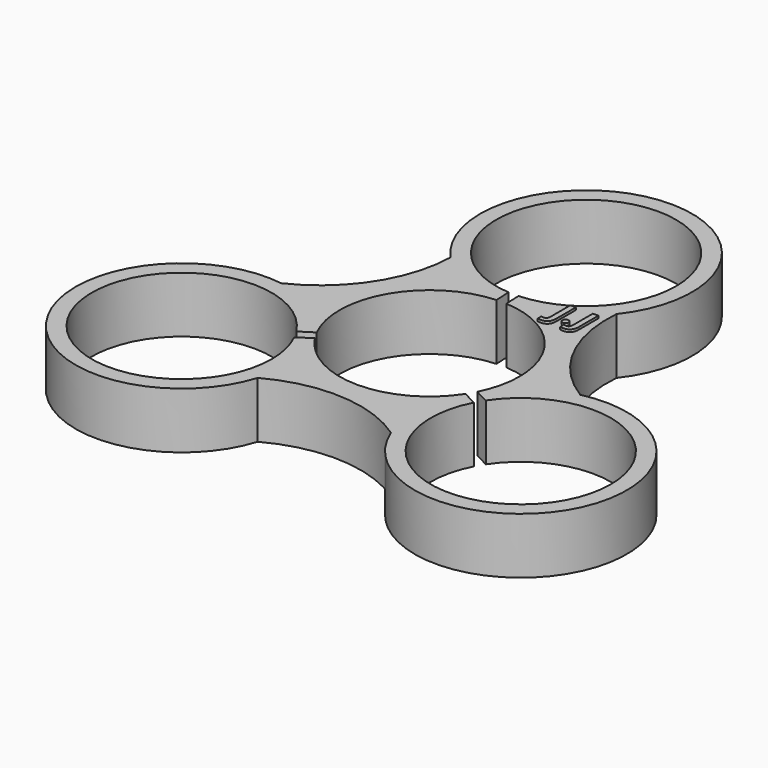
from build123d import *

# Parameters (mm, degrees)
F1_DEPTH     = 7
F2_TEXT_SIZE = 4.5465331318
F3_DEPTH     = 0.3


# Not quite as in the source:
# - Text() gives the source's letters only with a copy of the font that has no kerning and outlines rounded to 1/6400 em; it was checked with that copy


with BuildPart() as f1:
    # F0 (on Top) → F1 (new body)
    with BuildSketch(Plane.XY):
        with BuildLine():
            ThreePointArc((18.2079299196, 0.6939532345), (12.0807069533, 7.3130394607), (10.3395173195, 16.1630915739))
            ThreePointArc((10.3395173195, 16.1630915739), (-0.4879958353, 37.5598209951), (-9.7049460899, 15.4215532434))
            ThreePointArc((-9.7049460899, 15.4215532434), (-12.3736314285, 6.8056793869), (-19.1674065665, 0.8727388746))
            ThreePointArc((-19.1674065665, 0.8727388746), (-32.2837612257, -19.2025272879), (-8.5029838297, -16.1155064779))
            ThreePointArc((-8.5029838297, -16.1155064779), (0.2929244752, -14.1187188476), (8.827889247, -17.0358304485))
            ThreePointArc((8.827889247, -17.0358304485), (32.771757061, -18.3572937072), (18.2079299196, 0.6939532345))
        make_face()
        with BuildLine():
            ThreePointArc((0.6142437825, 11.1831437698), (8.1338653285, 7.6993658712), (11.2, 0))
            ThreePointArc((11.2, 0), (10.893816941, -2.6009137732), (9.99200849, -5.0596211652))
            Line((9.99200849, -5.0596211652), (11.7832934923, -5.9744533529))
            ThreePointArc((11.7832934923, -5.9744533529), (24.348083489, -1.4645262017), (32.3040384251, -12.1844222657))
            ThreePointArc((32.3040384251, -12.1844222657), (18.4597818184, -23.0677998204), (11.1526264612, -7.0454145867))
            Line((11.1526264612, -7.0454145867), (9.3777647076, -6.1235226046))
            ThreePointArc((9.3777647076, -6.1235226046), (0, -11.2), (-9.3777647076, -6.1235226046))
            Line((-9.3777647076, -6.1235226046), (-11.0656751235, -7.2174048282))
            ThreePointArc((-11.0656751235, -7.2174048282), (-10.1983135758, -9.6338996701), (-9.9040384251, -12.1844222657))
            ThreePointArc((-9.9040384251, -12.1844222657), (-31.8514481698, -15.3361176475), (-11.6778212429, -6.1357505409))
            Line((-11.6778212429, -6.1357505409), (-9.99200849, -5.0596211652))
            ThreePointArc((-9.99200849, -5.0596211652), (-9.6994845224, 5.6), (-0.6142437825, 11.1831437698))
            Line((-0.6142437825, 11.1831437698), (-0.7176183689, 13.191858181))
            ThreePointArc((-0.7176183689, 13.191858181), (-7.6616797854, 32.5382179998), (11.2, 24.3688445314))
            ThreePointArc((11.2, 24.3688445314), (8.103153138, 16.6371623586), (0.5251947817, 13.1811651277))
            Line((0.5251947817, 13.1811651277), (0.6142437825, 11.1831437698))
        make_face(mode=Mode.SUBTRACT)
    extrude(amount=F1_DEPTH)

    # F2 (on face) → F3 (join)
    with BuildSketch(Plane.XY.offset(7)):
        with Locations((5.6404429488, 11.1082233489)):
            Text('J.J', F2_TEXT_SIZE, font='Open Sans', font_style=FontStyle.BOLD, text_align=(TextAlign.LEFT, TextAlign.BOTTOM))
    extrude(amount=F3_DEPTH)


solid = f1.part
